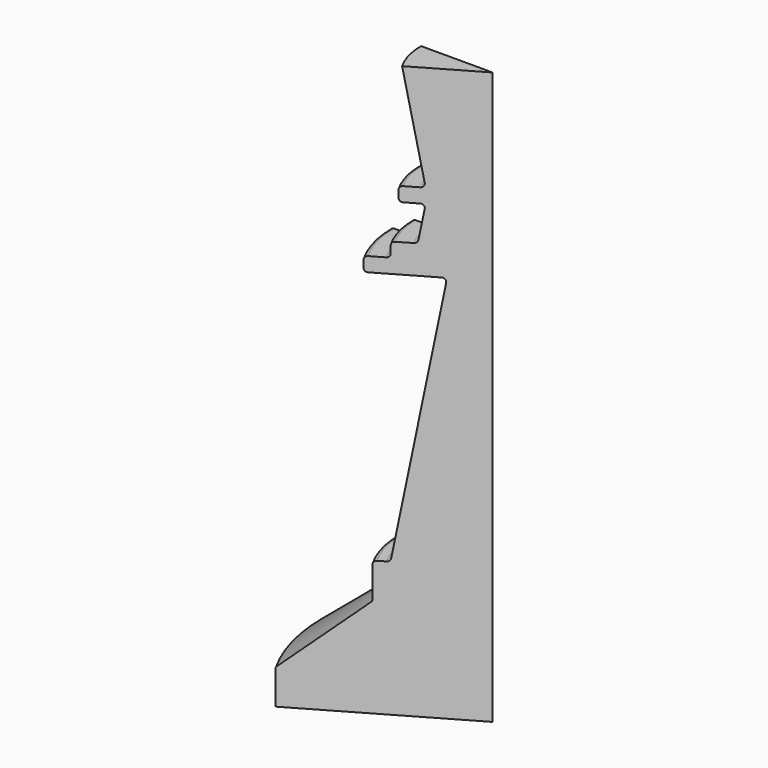
from build123d import *

# Parameters (mm, degrees)
F1_ANGLE = 30


# Not quite as in the source:
# - a feature of the source that left no trace in its solid (it failed there, or was rolled back) is left out


with BuildPart() as f1:
    # F0 (on Front) → F1 (revolve)
    with BuildSketch(Plane.XZ):
        with BuildLine():
            Line((-15.24, 0), (0, 0))
            Line((0, 0), (0, 50.8))
            Line((0, 50.8), (-6.35, 50.8))
            Line((-6.35, 50.8), (-4.7617064118, 41.792339449))
            ThreePointArc((-4.7617064118, 41.792339449), (-4.8311637627, 41.5331210865), (-5.0743828734, 41.4197061526))
            Line((-5.0743828734, 41.4197061526), (-6.2835011077, 41.4197061526))
            ThreePointArc((-6.2835011077, 41.4197061526), (-6.5080075107, 41.3267125556), (-6.6010011077, 41.1022061526))
            Line((-6.6010011077, 41.1022061526), (-6.6010011077, 40.4672061526))
            ThreePointArc((-6.6010011077, 40.4672061526), (-6.5080075107, 40.2426997495), (-6.2835011077, 40.1497061526))
            Line((-6.2835011077, 40.1497061526), (-5.0743828734, 40.1497061526))
            ThreePointArc((-5.0743828734, 40.1497061526), (-4.8311637627, 40.0362912186), (-4.7617064118, 39.7770728561))
            Line((-4.7617064118, 39.7770728561), (-5.2010717431, 37.2853082403))
            ThreePointArc((-5.2010717431, 37.2853082403), (-5.3096631386, 37.0972224261), (-5.5137482047, 37.0229415367))
            Line((-5.5137482047, 37.0229415367), (-6.8348340718, 37.0229415367))
            ThreePointArc((-6.8348340718, 37.0229415367), (-7.0593404748, 36.9299479398), (-7.1523340718, 36.7054415367))
            Line((-7.1523340718, 36.7054415367), (-7.1523340718, 36.0704415367))
            ThreePointArc((-7.1523340718, 36.0704415367), (-7.2453276688, 35.8459351337), (-7.4698340718, 35.7529415367))
            Line((-7.4698340718, 35.7529415367), (-8.7398340718, 35.7529415367))
            ThreePointArc((-8.7398340718, 35.7529415367), (-8.9643404748, 35.6599479398), (-9.0573340718, 35.4354415367))
            Line((-9.0573340718, 35.4354415367), (-9.0573340718, 34.8004415367))
            ThreePointArc((-9.0573340718, 34.8004415367), (-8.9643404748, 34.5759351337), (-8.7398340718, 34.4829415367))
            Line((-8.7398340718, 34.4829415367), (-3.5686493249, 34.4829415367))
            ThreePointArc((-3.5686493249, 34.4829415367), (-3.3254302142, 34.3695266028), (-3.2559728633, 34.1103082403))
            Line((-3.2559728633, 34.1103082403), (-7.113602572, 12.2326030065))
            ThreePointArc((-7.113602572, 12.2326030065), (-7.2221939675, 12.0445171922), (-7.4262790336, 11.9702363029))
            Line((-7.4262790336, 11.9702363029), (-8.1123649007, 11.9702363029))
            ThreePointArc((-8.1123649007, 11.9702363029), (-8.3368713037, 11.8772427059), (-8.4298649007, 11.6527363029))
            Line((-8.4298649007, 11.6527363029), (-8.4298649007, 8.9432889844))
            ThreePointArc((-8.4298649007, 8.9432889844), (-8.4596121783, 8.8091076862), (-8.5432798346, 8.7000698737))
            Line((-8.5432798346, 8.7000698737), (-15.1265850661, 3.176020882))
            ThreePointArc((-15.1265850661, 3.176020882), (-15.2102527224, 3.0669830694), (-15.24, 2.9328017713))
            Line((-15.24, 2.9328017713), (-15.24, 0))
        make_face()
    revolve(axis=Axis((0, 0, 25.4), (0, 0, 1)), revolution_arc=F1_ANGLE)


solid = f1.part
